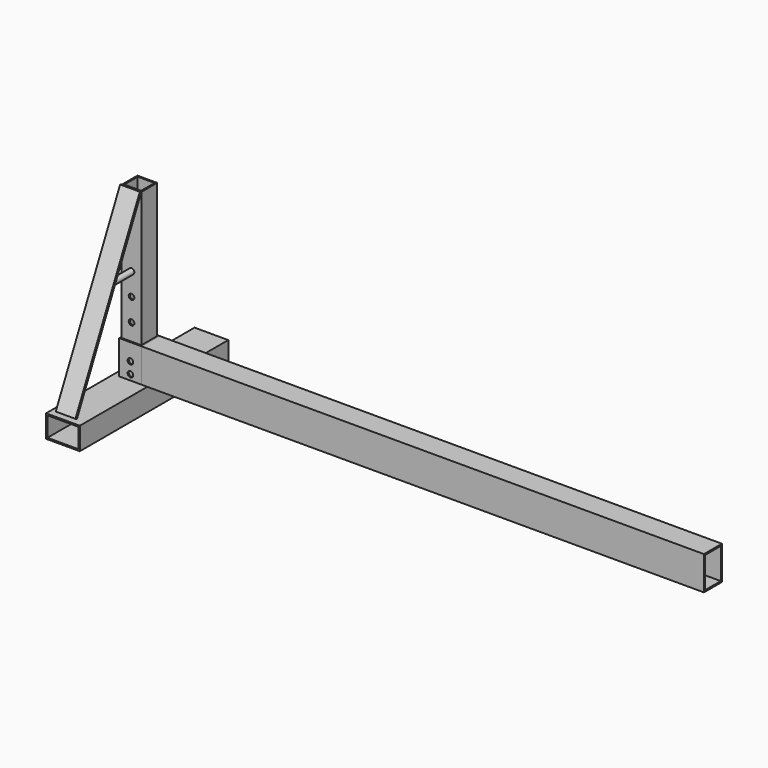
from build123d import *

# Parameters (mm, degrees)
F0_W           = 101.6
F0_H           = 101.6
F0_W_2         = 88.8999998569
F0_H_2         = 88.8999998569
F1_DEPTH       = 152.4
F2_W           = 88.8999998569
F2_H           = 88.8999998569
F2_W_2         = 76.1999998569
F2_H_2         = 76.1999998569
F3_DEPTH       = 762
F4_W           = 101.6
F4_H           = 152.4
F4_W_2         = 88.9
F4_H_2         = 139.7
F5_DEPTH       = 2540
F7_W           = 152.4
F7_H           = 101.6
F7_W_2         = 139.6999955177
F7_H_2         = 88.8999955177
F8_DEPTH       = 838.2
F12_W          = 88.9
F12_H          = 9.525
F13_DEPTH      = 838.2
F14_R          = 12.7
F15_DEPTH      = 482.601
F16_R          = 12.7
F17_DEPTH      = 476.2509999285
F18_DEPTH      = 233.68
F18_DEPTH_BACK = 25.4
F19_R          = 12.7
F20_DEPTH      = 482.601


with BuildPart() as f1:
    # F0 (on Top) → F1 (new body)
    with BuildSketch(Plane.XY):
        with Locations((-139.3107622862, 0)):
            Rectangle(F0_W, F0_H)
        with Locations((-139.3107622862, 0)):
            Rectangle(F0_W_2, F0_H_2, mode=Mode.SUBTRACT)
    extrude(amount=F1_DEPTH)

    # F14 (on face) → F15 (cut, through all)
    with BuildSketch(Plane(origin=(0, 50.8, 0), x_dir=(-1, 0, 0), z_dir=(0, 1, 0))):
        with Locations((139.3107622862, 25.4)):
            Circle(F14_R)
    extrude(amount=-F15_DEPTH, mode=Mode.SUBTRACT)

    # F19 (on face) → F20 (cut, through all)
    with BuildSketch(Plane(origin=(0, 50.8, 0), x_dir=(-1, 0, 0), z_dir=(0, 1, 0))):
        with Locations((139.3107622862, 76.2)):
            Circle(F19_R)
    extrude(amount=-F20_DEPTH, mode=Mode.SUBTRACT)


with BuildPart() as f3:
    # F2 (on face) → F3 (new body)
    with BuildSketch(Plane(origin=(0, 0, 0), x_dir=(1, 0, 0), z_dir=(0, 0, -1))):
        with Locations((-139.3107622862, 0)):
            Rectangle(F2_W, F2_H)
        with Locations((-139.3107622862, 0)):
            Rectangle(F2_W_2, F2_H_2, mode=Mode.SUBTRACT)
    extrude(amount=-F3_DEPTH)

    # F16 (on face) → F17 (cut, through all)
    with BuildSketch(Plane(origin=(0, 44.4499999285, 0), x_dir=(-1, 0, 0), z_dir=(0, 1, 0))):
        with Locations((139.3107622862, 431.8)):
            Circle(F16_R)
        with Locations((139.3107622862, 330.2)):
            Circle(F16_R)
        with Locations((139.3107622862, 228.6)):
            Circle(F16_R)
        with Locations((139.3107622862, 127)):
            Circle(F16_R)
    extrude(amount=-F17_DEPTH, mode=Mode.SUBTRACT)


with BuildPart() as f5:
    # F4 (on face) → F5 (new body)
    with BuildSketch(Plane.YZ.offset(-88.5107622862)):
        with Locations((0, 76.2)):
            Rectangle(F4_W, F4_H)
        with Locations((0, 76.2)):
            Rectangle(F4_W_2, F4_H_2, mode=Mode.SUBTRACT)
    extrude(amount=F5_DEPTH)


with BuildPart() as f8:
    # F7 (on offset) → F8 (new body)
    with BuildSketch(Plane.XZ.offset(431.8)):
        with Locations((-139.3107622862, -50.8)):
            Rectangle(F7_W, F7_H)
        with Locations((-139.3107622862, -50.8)):
            Rectangle(F7_W_2, F7_H_2, mode=Mode.SUBTRACT)
    extrude(amount=-F8_DEPTH)


with BuildPart() as f13:
    # F12 (on face) → F13 (new body)
    with BuildSketch(Plane(origin=(0, 289.5250416317, 601.1014136742), x_dir=(1, 0, 0), z_dir=(0, 0.4339443975, 0.9009396539))):
        with Locations((-139.4686400175, -375.4748984393)):
            Rectangle(F12_W, F12_H)
    extrude(amount=-F13_DEPTH)


with BuildPart() as f18:
    # F16 (on face) → F18 (new body, two sides)
    with BuildSketch(Plane(origin=(0, 44.4499999285, 0), x_dir=(-1, 0, 0), z_dir=(0, 1, 0))) as f18_sk:
        with Locations((139.3107622862, 431.8)):
            Circle(F16_R)
    extrude(amount=-F18_DEPTH)
    extrude(f18_sk.sketch, amount=F18_DEPTH_BACK)


solid = Compound([f1.part, f3.part, f5.part, f8.part, f13.part, f18.part])
